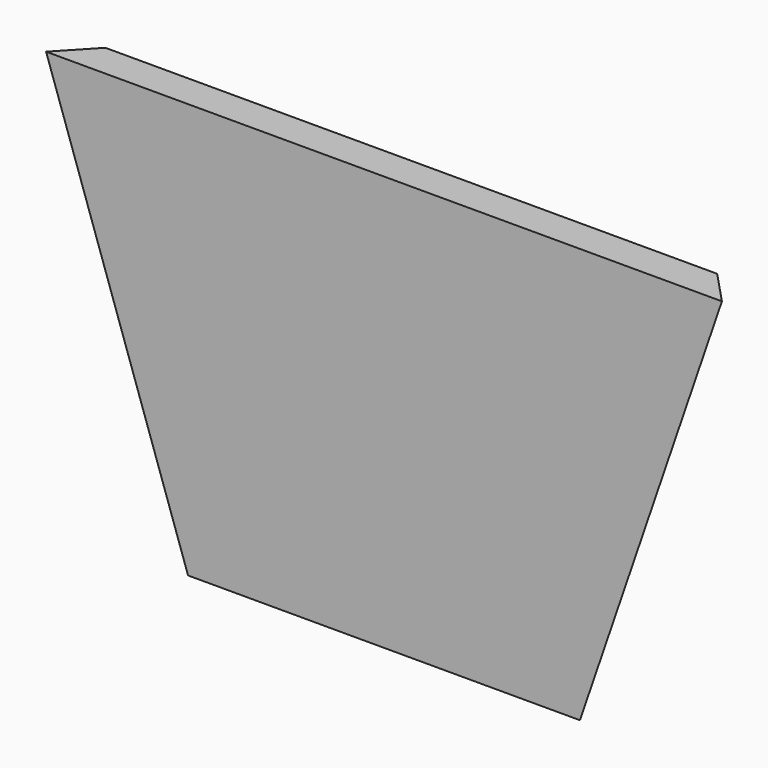
from build123d import *

# Parameters (mm, degrees)
F0_W     = 115
F0_H     = 121.7650999273
F1_DEPTH = 10
F2_SIZE2 = 8.888878
F2_SIZE  = 9.99999
F3_SIZE2 = 9.99999
F3_SIZE  = 8.888878


# Not quite as in the source:
# - a fillet or chamfer is up to 0.001 mm smaller than in the source, because OpenCascade refuses the exact size


with BuildPart() as f1:
    # F0 (on Front) → F1 (new body)
    with BuildSketch(Plane.XZ):
        with Locations((-35.6102311611, 0.0679380756)):
            Rectangle(F0_W, F0_H)
        Polygon((-93.1102311611, -60.814611888), (-93.1102311611, 60.9504880392), (-134.7733613184, 60.9504880392), align=None)
        Polygon((63.5528989962, 60.9504880392), (21.8897688389, 60.9504880392), (21.8897688389, -60.814611888), align=None)
    extrude(amount=F1_DEPTH)

    # F2 (size 10 and 8.888888 in the source; OpenCascade refuses exactly that, so slightly less here)
    f2_edges = [f1.edges().sort_by_distance(p)[0] for p in [
        (-113.941796, 0, 0.067938),
    ]]
    f2_side = f1.faces().sort_by_distance((-113.941796, -5, 0.067938))[0]
    chamfer(f2_edges, length=F2_SIZE, length2=F2_SIZE2, reference=f2_side)

    # F3 (size 8.888888 and 10 in the source; OpenCascade refuses exactly that, so slightly less here)
    f3_edges = [f1.edges().sort_by_distance(p)[0] for p in [
        (42.721334, 0, 0.067938),
    ]]
    f3_side = f1.faces().sort_by_distance((-30.912828, 0, 5.809289))[0]
    chamfer(f3_edges, length=F3_SIZE, length2=F3_SIZE2, reference=f3_side)


solid = f1.part
